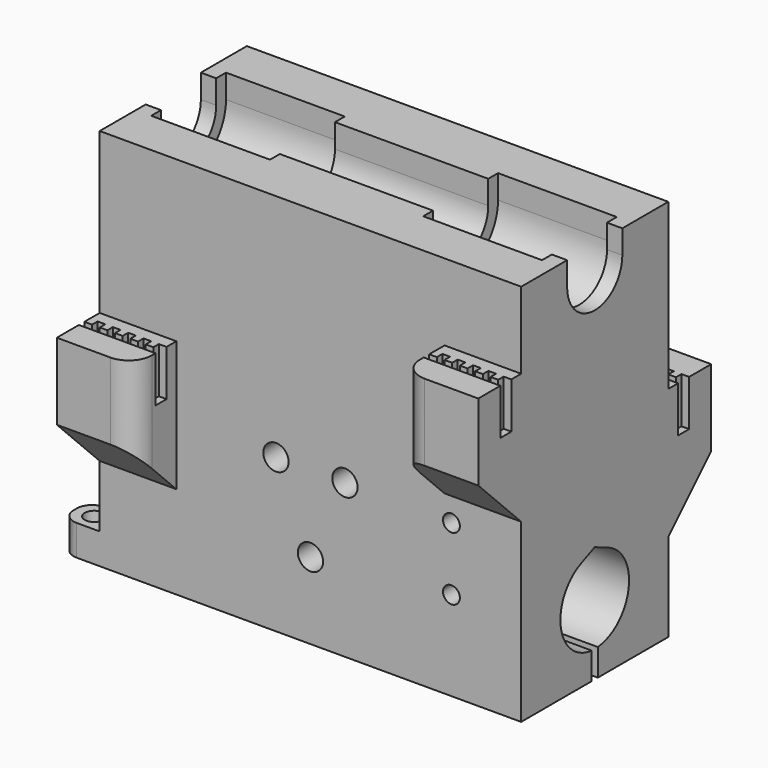
from build123d import *

# Parameters (mm, degrees)
F0_W         = 55
F0_H         = 24
F1_DEPTH     = 50
F1_FACE1_W   = 24
F1_FACE1_H   = 50
F3_DEPTH     = 55.001
F4_DEPTH     = 53
F5_DEPTH     = 2
F6_START     = 15.5
F6_DEPTH     = 20
F7_DEPTH     = 22.5
F8_START     = -32.5
F8_DEPTH     = 22.5
F9_W         = 10
F9_H         = 20
F10_DEPTH    = 7
F11_T4_DEPTH = 61.4336597593
F11_T9_DEPTH = 61.4336597593
F13_DEPTH    = 6
F15_DEPTH    = 6
F16_W        = 10
F16_H        = 20
F17_DEPTH    = 7
F19_DEPTH    = 6
F21_DEPTH    = 6
F22_T4_DEPTH = 61.4336597593
F22_T9_DEPTH = 61.4336597593
F23_R        = 1.65
F24_DEPTH    = 31.001
F25_R        = 1.1
F26_DEPTH    = 5
F27_W        = 4.5
F27_H        = 4
F28_DEPTH    = 5
F29_R        = 1.25
F30_DEPTH    = 25
F31_R        = 2
F32_R        = 3


# Not quite as in the source:
# - a fillet or chamfer that OpenCascade refuses, or shapes differently, is made with other operations: its cross-section is extruded or revolved along the edge and cut away or added
# - a feature names something its author has since deleted; it is built from what else it names


with BuildPart() as f1:
    # F0 (on Top) → F1 (new body)
    with BuildSketch(Plane.XY):
        with Locations((27.5, 12)):
            Rectangle(F0_W, F0_H)
    extrude(amount=F1_DEPTH)

    # F2 (on face) + F1_face1 (on face) → F3 (cut, through all)
    with BuildSketch(Plane(origin=(0, 0, 0), x_dir=(0, -1, 0), z_dir=(-1, 0, 0))):
        with BuildLine():
            Line((-11.5, 0), (-11.5, 3.522366093))
            ThreePointArc((-11.5, 3.522366093), (-12, 3.5), (-12.5, 3.522366093))
            Line((-12.5, 3.522366093), (-12.5, 0))
            Line((-12.5, 0), (-12, 0))
            Line((-12, 0), (-11.5, 0))
        make_face()
        with BuildLine():
            ThreePointArc((-12.5, 4.627864045), (-12, 4.6), (-11.5, 4.627864045))
            Line((-11.5, 4.627864045), (-12.5, 4.627864045))
        make_face()
        with BuildLine():
            Line((-7.5, 46.9), (-7.5, 50))
            Line((-7.5, 50), (-8.7380987139, 50))
            ThreePointArc((-8.7380987139, 50), (-7.8209716568, 48.5690482636), (-7.5, 46.9))
        make_face()
        with BuildLine():
            Line((-15.2619012861, 50), (-16.5, 50))
            Line((-16.5, 50), (-16.5, 46.9))
            ThreePointArc((-16.5, 46.9), (-16.1790283432, 48.5690482636), (-15.2619012861, 50))
        make_face()
        with BuildLine():
            ThreePointArc((-16.5, 46.9), (-12, 42.4), (-7.5, 46.9))
            ThreePointArc((-7.5, 46.9), (-7.8209716568, 48.5690482636), (-8.7380987139, 50))
            Line((-8.7380987139, 50), (-15.2619012861, 50))
            ThreePointArc((-15.2619012861, 50), (-16.1790283432, 48.5690482636), (-16.5, 46.9))
        make_face()
        with BuildLine():
            Line((-12.5, 4.627864045), (-11.5, 4.627864045))
            ThreePointArc((-11.5, 4.627864045), (-8.6458980338, 6.1), (-7.5, 9.1))
            ThreePointArc((-7.5, 9.1), (-15, 12.4541019662), (-12.5, 4.627864045))
        make_face()
        with BuildLine():
            ThreePointArc((-12.5, 3.522366093), (-12, 3.5), (-11.5, 3.522366093))
            Line((-11.5, 3.522366093), (-11.5, 4.627864045))
            ThreePointArc((-11.5, 4.627864045), (-12, 4.6), (-12.5, 4.627864045))
            Line((-12.5, 4.627864045), (-12.5, 3.522366093))
        make_face()
    with BuildSketch(Plane(origin=(55, 12, 25), x_dir=(0, 1, 0), z_dir=(1, 0, 0))):
        Rectangle(F1_FACE1_W, F1_FACE1_H)
    extrude(amount=-F3_DEPTH, dir=(-1, 0, 0), mode=Mode.SUBTRACT)

    # F2 (on face) → F4 (cut)
    with BuildSketch(Plane(origin=(0, 0, 0), x_dir=(0, -1, 0), z_dir=(-1, 0, 0))):
        with BuildLine():
            ThreePointArc((-18.1, 46.9), (-12, 40.8), (-5.9, 46.9))
            ThreePointArc((-5.9, 46.9), (-6.1154108763, 48.5067391964), (-6.7464297854, 50))
            Line((-6.7464297854, 50), (-7.5, 50))
            Line((-7.5, 50), (-7.5, 46.9))
            ThreePointArc((-7.5, 46.9), (-12, 42.4), (-16.5, 46.9))
            Line((-16.5, 46.9), (-16.5, 50))
            Line((-16.5, 50), (-17.2535702146, 50))
            ThreePointArc((-17.2535702146, 50), (-17.8845891237, 48.5067391964), (-18.1, 46.9))
        make_face()
        with BuildLine():
            Line((-17.2535702146, 50), (-18.1, 50))
            Line((-18.1, 50), (-18.1, 46.9))
            ThreePointArc((-18.1, 46.9), (-17.8845891237, 48.5067391964), (-17.2535702146, 50))
        make_face()
        with BuildLine():
            Line((-5.9, 46.9), (-5.9, 50))
            Line((-5.9, 50), (-6.7464297854, 50))
            ThreePointArc((-6.7464297854, 50), (-6.1154108763, 48.5067391964), (-5.9, 46.9))
        make_face()
    extrude(amount=-F4_DEPTH, mode=Mode.SUBTRACT)

    # F2 (on face) → F5 (join)
    with BuildSketch(Plane(origin=(0, 0, 0), x_dir=(0, -1, 0), z_dir=(-1, 0, 0))):
        with BuildLine():
            ThreePointArc((-18.1, 46.9), (-12, 40.8), (-5.9, 46.9))
            ThreePointArc((-5.9, 46.9), (-6.1154108763, 48.5067391964), (-6.7464297854, 50))
            Line((-6.7464297854, 50), (-7.5, 50))
            Line((-7.5, 50), (-7.5, 46.9))
            ThreePointArc((-7.5, 46.9), (-12, 42.4), (-16.5, 46.9))
            Line((-16.5, 46.9), (-16.5, 50))
            Line((-16.5, 50), (-17.2535702146, 50))
            ThreePointArc((-17.2535702146, 50), (-17.8845891237, 48.5067391964), (-18.1, 46.9))
        make_face()
        with BuildLine():
            Line((-17.2535702146, 50), (-18.1, 50))
            Line((-18.1, 50), (-18.1, 46.9))
            ThreePointArc((-18.1, 46.9), (-17.8845891237, 48.5067391964), (-17.2535702146, 50))
        make_face()
        with BuildLine():
            Line((-5.9, 46.9), (-5.9, 50))
            Line((-5.9, 50), (-6.7464297854, 50))
            ThreePointArc((-6.7464297854, 50), (-6.1154108763, 48.5067391964), (-5.9, 46.9))
        make_face()
    extrude(amount=-F5_DEPTH)

    # F5_face (on face) → F6 (join)
    with BuildSketch(Plane(origin=(2, 12, 44.8432927997), x_dir=(0, 1, 0), z_dir=(1, 0, 0)).offset(F6_START)):
        with BuildLine():
            ThreePointArc((-6.1, 2.0567072003), (0, -4.0432927997), (6.1, 2.0567072003))
            Line((6.1, 2.0567072003), (6.1, 5.1567072003))
            Line((6.1, 5.1567072003), (4.5, 5.1567072003))
            Line((4.5, 5.1567072003), (4.5, 2.0567072003))
            ThreePointArc((4.5, 2.0567072003), (0, -2.4432927997), (-4.5, 2.0567072003))
            Line((-4.5, 2.0567072003), (-4.5, 5.1567072003))
            Line((-4.5, 5.1567072003), (-6.1, 5.1567072003))
            Line((-6.1, 5.1567072003), (-6.1, 2.0567072003))
        make_face()
    extrude(amount=F6_DEPTH)

    # F2 (on face) → F7 (cut)
    with BuildSketch(Plane(origin=(0, 0, 0), x_dir=(0, -1, 0), z_dir=(-1, 0, 0))):
        with BuildLine():
            ThreePointArc((-11.5, 3.522366093), (-7.867204336, 5.3211112745), (-6.4, 9.1))
            ThreePointArc((-6.4, 9.1), (-7.3061186168, 12.1540919372), (-9.731241986, 14.2198376023))
            Line((-9.731241986, 14.2198376023), (-12, 15.2))
            Line((-12, 15.2), (-14.268758014, 14.2198376023))
            ThreePointArc((-14.268758014, 14.2198376023), (-17.5249868242, 8.1864790138), (-12.5, 3.522366093))
            Line((-12.5, 3.522366093), (-12.5, 4.627864045))
            ThreePointArc((-12.5, 4.627864045), (-15, 12.4541019662), (-7.5, 9.1))
            ThreePointArc((-7.5, 9.1), (-8.6458980338, 6.1), (-11.5, 4.627864045))
            Line((-11.5, 4.627864045), (-11.5, 3.522366093))
        make_face()
        with BuildLine():
            Line((-12.5, 4.627864045), (-11.5, 4.627864045))
            ThreePointArc((-11.5, 4.627864045), (-8.6458980338, 6.1), (-7.5, 9.1))
            ThreePointArc((-7.5, 9.1), (-15, 12.4541019662), (-12.5, 4.627864045))
        make_face()
    extrude(amount=-F7_DEPTH, mode=Mode.SUBTRACT)

    # F2 (on face) → F8 (cut)
    with BuildSketch(Plane(origin=(0, 0, 0), x_dir=(0, -1, 0), z_dir=(-1, 0, 0)).offset(F8_START)):
        with BuildLine():
            ThreePointArc((-11.5, 3.522366093), (-7.867204336, 5.3211112745), (-6.4, 9.1))
            ThreePointArc((-6.4, 9.1), (-7.3061186168, 12.1540919372), (-9.731241986, 14.2198376023))
            Line((-9.731241986, 14.2198376023), (-12, 15.2))
            Line((-12, 15.2), (-14.268758014, 14.2198376023))
            ThreePointArc((-14.268758014, 14.2198376023), (-17.5249868242, 8.1864790138), (-12.5, 3.522366093))
            Line((-12.5, 3.522366093), (-12.5, 4.627864045))
            ThreePointArc((-12.5, 4.627864045), (-15, 12.4541019662), (-7.5, 9.1))
            ThreePointArc((-7.5, 9.1), (-8.6458980338, 6.1), (-11.5, 4.627864045))
            Line((-11.5, 4.627864045), (-11.5, 3.522366093))
        make_face()
        with BuildLine():
            Line((-12.5, 4.627864045), (-11.5, 4.627864045))
            ThreePointArc((-11.5, 4.627864045), (-8.6458980338, 6.1), (-7.5, 9.1))
            ThreePointArc((-7.5, 9.1), (-15, 12.4541019662), (-12.5, 4.627864045))
        make_face()
    extrude(amount=-F8_DEPTH, mode=Mode.SUBTRACT)

    # F9 (on face) → F10 (join)
    with BuildSketch(Plane.XZ):
        with Locations((5, 19.1)):
            Rectangle(F9_W, F9_H)
        with Locations((50, 30)):
            Rectangle(F9_W, F9_H)
    extrude(amount=F10_DEPTH)

    # F11: chamfer of 10 on 2 edges, made by hand


with BuildPart() as f11_tool2:
    # F11_s3 → F11_t4 (new body)
    with BuildSketch(Plane.YZ.offset(-25.7168298797)):
        Polygon((3, 9.1), (-7, 19.1), (-7, 9.1), align=None)
    extrude(amount=F11_T4_DEPTH)

    split(bisect_by=Plane.XZ, keep=Keep.TOP)


with BuildPart() as f1_1:
    add(f1.part)

    # F11_t1: cut F11_tool2
    add(f11_tool2.part, mode=Mode.SUBTRACT)


with BuildPart() as f11_tool7:
    # F11_s8 → F11_t9 (new body)
    with BuildSketch(Plane.YZ.offset(19.2831701203)):
        Polygon((3, 20), (-7, 30), (-7, 20), align=None)
    extrude(amount=F11_T9_DEPTH)

    split(bisect_by=Plane.XZ, keep=Keep.TOP)


with BuildPart() as f1_2:
    add(f1_1.part)

    # F11_t6: cut F11_tool7
    add(f11_tool7.part, mode=Mode.SUBTRACT)

    # F12 (on face) → F13 (cut)
    with BuildSketch(Plane.XY.offset(29.1)):
        Polygon((0, -2.5), (0, -3.4), (10, -3.4), (10, -2.5), (10, -1.6), (9, -1.6), (9, -2.5), (8, -2.5), (8, -1.6), (7, -1.6), (7, -2.5), (6, -2.5), (6, -1.6), (5.2958247252, -1.6), (5, -1.6), (5, -2.5), (4, -2.5), (4, -1.6), (3, -1.6), (3, -2.5), (2, -2.5), (2, -1.6), (1, -1.6), (1, -2.5), align=None)
    extrude(amount=-F13_DEPTH, mode=Mode.SUBTRACT)

    # F14 (on face) → F15 (cut)
    with BuildSketch(Plane.XY.offset(40)):
        Polygon((45, -2.5), (45, -3.4), (55, -3.4), (55, -2.5), (55, -1.6), (54, -1.6), (54, -2.5), (53, -2.5), (53, -1.6), (52, -1.6), (52, -2.5), (51, -2.5), (51, -1.6), (50.2349036932, -1.6), (50, -1.6), (50, -2.5), (49, -2.5), (49, -1.6), (48, -1.6), (48, -2.5), (47, -2.5), (47, -1.6), (46, -1.6), (46, -2.5), align=None)
    extrude(amount=-F15_DEPTH, mode=Mode.SUBTRACT)

    # F16 (on face) → F17 (join)
    with BuildSketch(Plane(origin=(0, 24, 0), x_dir=(-1, 0, 0), z_dir=(0, 1, 0))):
        with Locations((-50, 18.5)):
            Rectangle(F16_W, F16_H)
        with Locations((-5, 30)):
            Rectangle(F16_W, F16_H)
    extrude(amount=F17_DEPTH)

    # F18 (on face) → F19 (cut)
    with BuildSketch(Plane.XY.offset(28.5)):
        Polygon((45, 26.5), (45, 25.6), (50, 25.6), (55, 25.6), (55, 26.5), (55, 27.4), (54, 27.4), (54, 26.5), (53, 26.5), (53, 27.4), (52, 27.4), (52, 26.5), (51, 26.5), (51, 27.4), (50, 27.4), (50, 26.5), (49, 26.5), (49, 27.4), (48, 27.4), (48, 26.5), (47, 26.5), (47, 27.4), (46, 27.4), (46, 26.5), align=None)
    extrude(amount=-F19_DEPTH, mode=Mode.SUBTRACT)

    # F20 (on face) → F21 (cut)
    with BuildSketch(Plane.XY.offset(40)):
        Polygon((7, 26.5), (6, 26.5), (6, 27.4), (5, 27.4), (5, 26.5), (4, 26.5), (4, 27.4), (3, 27.4), (3, 26.5), (2, 26.5), (2, 27.4), (1, 27.4), (1, 26.5), (0, 26.5), (0, 25.6), (5, 25.6), (10, 25.6), (10, 26.5), (10, 27.4), (9, 27.4), (9, 26.5), (8, 26.5), (8, 27.4), (7, 27.4), align=None)
    extrude(amount=-F21_DEPTH, mode=Mode.SUBTRACT)

    # F22: chamfer of 10 on 2 edges, made by hand


with BuildPart() as f22_tool2:
    # F22_s3 → F22_t4 (new body)
    with BuildSketch(Plane.YZ.offset(35.7168298797)):
        Polygon((31, 30), (21, 20), (31, 20), align=None)
    extrude(amount=-F22_T4_DEPTH)

    split(bisect_by=Plane.XZ.offset(-24), keep=Keep.BOTTOM)


with BuildPart() as f1_3:
    add(f1_2.part)

    # F22_t1: cut F22_tool2
    add(f22_tool2.part, mode=Mode.SUBTRACT)


with BuildPart() as f22_tool7:
    # F22_s8 → F22_t9 (new body)
    with BuildSketch(Plane.YZ.offset(80.7168298797)):
        Polygon((21, 8.5), (31, 18.5), (31, 8.5), align=None)
    extrude(amount=-F22_T9_DEPTH)

    split(bisect_by=Plane.XZ.offset(-24), keep=Keep.BOTTOM)


with BuildPart() as f1_4:
    add(f1_3.part)

    # F22_t6: cut F22_tool7
    add(f22_tool7.part, mode=Mode.SUBTRACT)

    # F23 (on face) → F24 (cut, through all)
    with BuildSketch(Plane.XZ):
        with Locations((32, 20)):
            Circle(F23_R)
        with Locations((27.5, 10)):
            Circle(F23_R)
        with Locations((23, 20)):
            Circle(F23_R)
    extrude(amount=-F24_DEPTH, mode=Mode.SUBTRACT)

    # F25 (on face) → F26 (cut)
    with BuildSketch(Plane.XZ):
        with Locations((45.9, 19.9)):
            Circle(F25_R)
        with Locations((45.9, 11.65)):
            Circle(F25_R)
    extrude(amount=-F26_DEPTH, mode=Mode.SUBTRACT)

    # F27 (on face) → F28 (join)
    with BuildSketch(Plane(origin=(0, 0, 0), x_dir=(0, -1, 0), z_dir=(-1, 0, 0))):
        with Locations((-2.25, 2)):
            Rectangle(F27_W, F27_H)
        with Locations((-21.25, 2)):
            Rectangle(F27_W, F27_H)
    extrude(amount=F28_DEPTH)

    # F29 (on face) → F30 (cut)
    with BuildSketch(Plane.XY.offset(4)):
        with Locations((-2.5, 2.25)):
            Circle(F29_R)
        with Locations((-2.5, 21.25)):
            Circle(F29_R)
    extrude(amount=-F30_DEPTH, mode=Mode.SUBTRACT)

    # F31
    f31_edges = [f1_4.edges().sort_by_distance(p)[0] for p in [
        (-5, 4.5, 2),
        (-5, 0, 2),
        (-5, 19, 2),
        (-5, 23.5, 2),
    ]]
    fillet(f31_edges, radius=F31_R)

    # F32
    f32_edges = [f1_4.edges().sort_by_distance(p)[0] for p in [
        (10, -7, 24.1),
        (45, -7, 35),
        (10, 31, 35),
        (45, 31, 23.5),
    ]]
    fillet(f32_edges, radius=F32_R)


solid = f1_4.part
